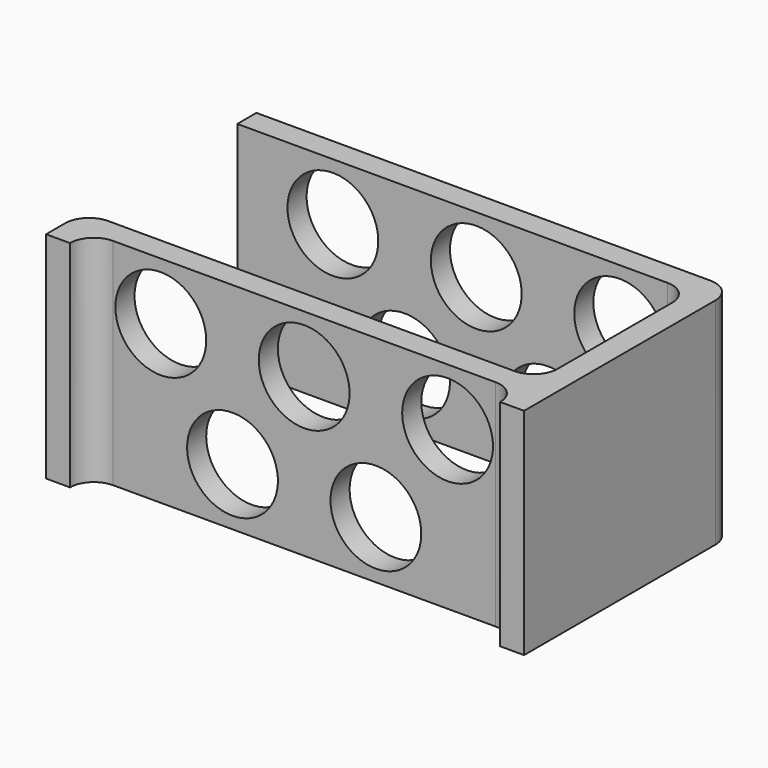
from build123d import *

# Parameters (mm, degrees)
F1_DEPTH = 45
F2_R     = 4.99999
F3_R     = 9.5
F4_DEPTH = 80


# Not quite as in the source:
# - a fillet or chamfer is up to 0.001 mm smaller than in the source, because OpenCascade refuses the exact size


with BuildPart() as f1:
    # F0 (on Top) → F1 (new body)
    with BuildSketch(Plane.XY):
        Polygon((65.8763971276, 17.5545628369), (-34.1236028724, 17.5545628369), (-34.1236028724, 12.5545628369), (60.8763971276, 12.5545628369), (60.8763971276, -27.4454371631), (-34.1236028724, -27.4454371631), (-34.1236028724, -32.4454371631), (-34.1236028724, -37.4454371631), (-29.1236028724, -37.4454371631), (-29.1236028724, -32.4454371631), (60.8763971276, -32.4454371631), (60.8763971276, -37.4454371631), (65.8763971276, -37.4454371631), (65.8763971276, -32.4454371631), align=None)
    extrude(amount=F1_DEPTH)

    # F2 (radius 5 in the source; OpenCascade refuses exactly that, so slightly less here)
    f2_edges = [f1.edges().sort_by_distance(p)[0] for p in [
        (60.876397, 12.554563, 22.5),
        (60.876397, -27.445437, 22.5),
        (65.876397, 17.554563, 22.5),
        (60.876397, -32.445437, 22.5),
        (-29.123603, -32.445437, 22.5),
        (-34.123603, -27.445437, 22.5),
    ]]
    fillet(f2_edges, radius=F2_R)

    # F3 (on face) → F4 (cut)
    with BuildSketch(Plane(origin=(0, 17.5545628369, 0), x_dir=(-1, 0, 0), z_dir=(0, 1, 0))):
        with Locations((-45.8763971276, 33)):
            Circle(F3_R)
        with Locations((-0.8763971276, 12)):
            Circle(F3_R)
        with Locations((14.1236028724, 33)):
            Circle(F3_R)
        with Locations((-30.8763971276, 12)):
            Circle(F3_R)
        with Locations((-15.8763971276, 33)):
            Circle(F3_R)
    extrude(amount=-F4_DEPTH, mode=Mode.SUBTRACT)


solid = f1.part
